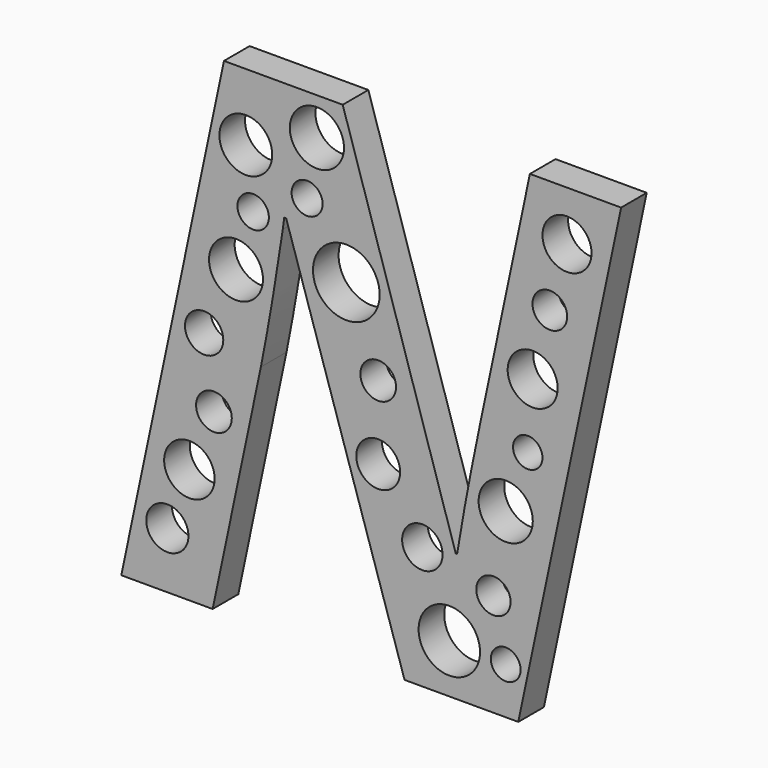
from build123d import *

# Parameters (mm, degrees)
F0_TEXT_SIZE = 75.5952386599
F1_DEPTH     = 3.556
F2_R         = 3.0059162341
F3_DEPTH     = 54.864
F4_R         = 2.7214288712
F4_R_2       = 1.9243405459
F4_R_3       = 2.7753238477
F4_R_4       = 1.6328576021
F4_R_5       = 3.005915138
F4_R_6       = 1.9049998373
F4_R_7       = 3.4099388626
F4_R_8       = 1.6553809547
F4_R_9       = 2.2441480087
F4_R_10      = 2.4341198245
F4_R_11      = 1.9812296153
F4_R_12      = 3.7015435389
F4_R_13      = 2.3410613309
F4_R_14      = 2.8018834882
F4_R_15      = 1.9812305587
F4_R_16      = 2.1255029181
F4_R_17      = 2.9935713392
F4_R_18      = 2.9310678009
F4_R_19      = 1.7425644693
F4_R_20      = 1.7211820083
F5_DEPTH     = 59.436


# Not quite as in the source:
# - Text() gives the source's letters only with a copy of the font that has no kerning and outlines rounded to 1/6400 em; it was checked with that copy


with BuildPart() as f1:
    # F0 (on Front) → F1 (new body)
    with BuildSketch(Plane.XZ):
        with Locations((-30.4800011218, -34.0178571641)):
            Text('N', F0_TEXT_SIZE, font='Open Sans', font_style=FontStyle.BOLDITALIC, text_align=(TextAlign.LEFT, TextAlign.BOTTOM))
    extrude(amount=F1_DEPTH)

    # F2 (on Front) → F3 (cut)
    with BuildSketch(Plane.XZ):
        with Locations((-6.8035717122, 15.7842859626)):
            Circle(F2_R)
    extrude(amount=F3_DEPTH, mode=Mode.SUBTRACT)

    # F4 (on Front) → F5 (cut)
    with BuildSketch(Plane.XZ):
        with Locations((20.9550019354, 14.423571527)):
            Circle(F4_R)
        with Locations((19.0500002354, 7.3478571139)):
            Circle(F4_R_2)
        with Locations((17.1449985355, 0)):
            Circle(F4_R_3)
        with Locations((16.6007149965, -7.3478571139)):
            Circle(F4_R_4)
        with Locations((14.1514278948, -13.8792861253)):
            Circle(F4_R_5)
        with Locations((12.7907134593, -22.5878581405)):
            Circle(F4_R_6)
        with Locations((7.89214205, -28.5750012845)):
            Circle(F4_R_7)
        with Locations((14.1514278948, -28.847143054)):
            Circle(F4_R_8)
        with Locations((4.8985718749, -20.410714671)):
            Circle(F4_R_9)
        with Locations((0, -13.8792861253)):
            Circle(F4_R_10)
        with Locations((0, -5.7150004432)):
            Circle(F4_R_11)
        with Locations((-3.5378576722, 2.7214286383)):
            Circle(F4_R_12)
        with Locations((-23.4042853117, -27.7585722506)):
            Circle(F4_R_13)
        with Locations((-20.9550000727, -21.2271418422)):
            Circle(F4_R_14)
        with Locations((-18.2335712016, -14.6957142279)):
            Circle(F4_R_15)
        with Locations((-19.322142005, -7.3478571139)):
            Circle(F4_R_16)
        with Locations((-15.7842859626, 0)):
            Circle(F4_R_17)
        with Locations((-14.6957151592, 12.5185707584)):
            Circle(F4_R_18)
        with Locations((-13.879285194, 6.2592853792)):
            Circle(F4_R_19)
        with Locations((-7.8921429813, 9.5250001177)):
            Circle(F4_R_20)
    extrude(amount=F5_DEPTH, mode=Mode.SUBTRACT)


solid = f1.part
